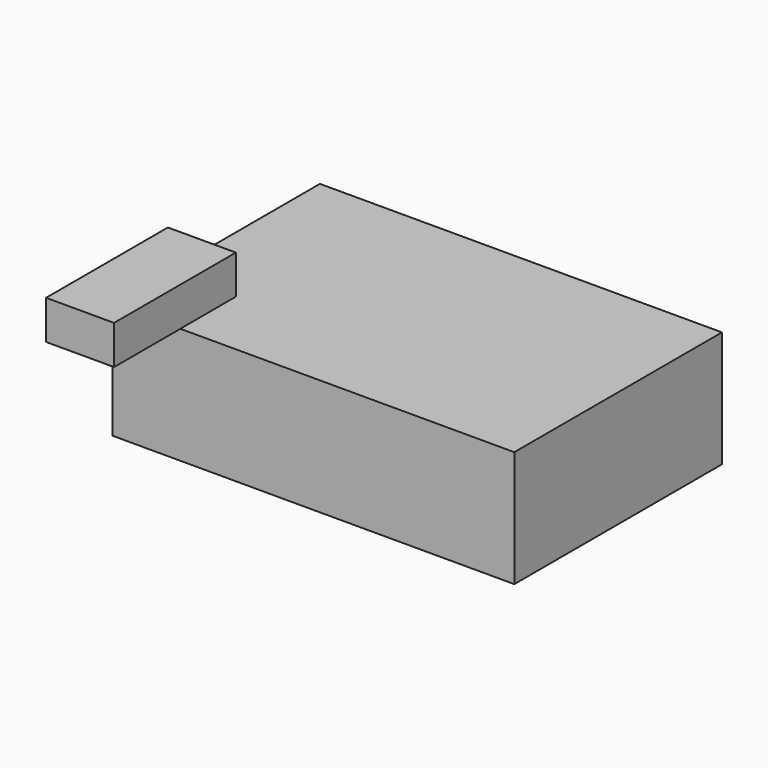
from build123d import *

# Parameters (mm, degrees)
F0_W     = 52.7686178684
F0_H     = 46.8310452998
F1_DEPTH = 45.0226236135
F2_W     = 61.3688528538
F2_H     = 15.6810022891
F3_DEPTH = 27.3912083358
F4_DEPTH = 109.2513594776
F5_DEPTH = 59.5592800528


# Not quite as in the source:
# - a feature names something its author has since deleted; it is built from what else it names


with BuildPart() as f1:
    # F0 (on Front) → F1 (new body)
    with BuildSketch(Plane.XZ):
        with Locations((26.3843089342, 23.4155226499)):
            Rectangle(F0_W, F0_H)
    extrude(amount=F1_DEPTH)

    # F2 (on Right) → F3 (join)
    with BuildSketch(Plane.YZ):
        with Locations((-47.6985424757, 54.6393077821)):
            Rectangle(F2_W, F2_H)
    extrude(amount=F3_DEPTH)

    # F4 (add): a face of the model
    f4_faces = [f1.faces().sort_by_distance(p)[0] for p in [
        (52.7686178684, -22.5113118067, 23.4155226499),
    ]]
    extrude(f4_faces, amount=F4_DEPTH)

    # F5 (add): a face of the model
    f5_faces = [f1.faces().sort_by_distance(p)[0] for p in [
        (81.009988673, 0, 23.4155226499),
    ]]
    extrude(f5_faces, amount=F5_DEPTH)


solid = f1.part
